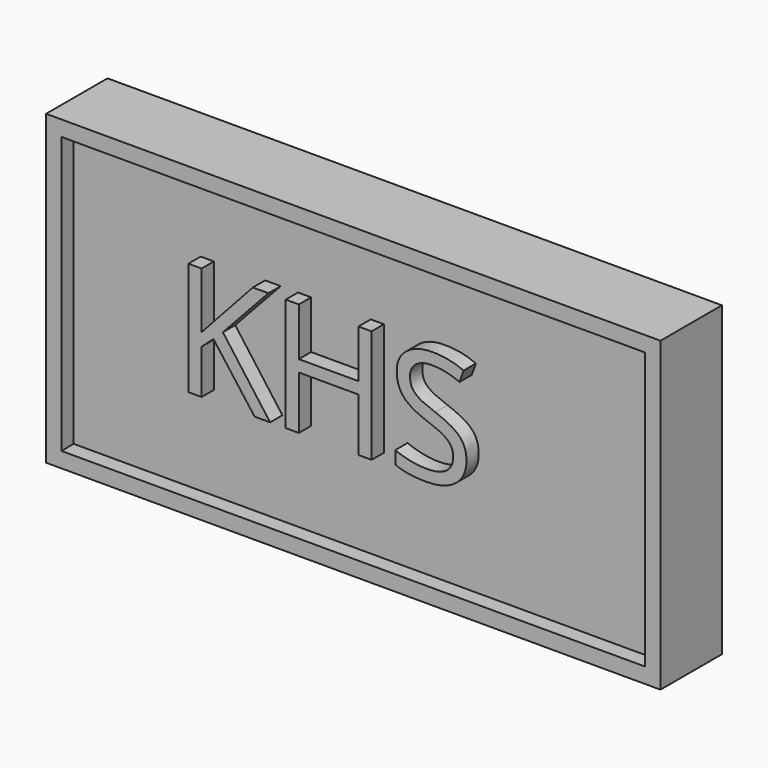
from build123d import *

# Parameters (mm, degrees)
F0_W         = 200
F0_H         = 100
F1_DEPTH     = 25
F2_W         = 190
F2_H         = 90
F3_DEPTH     = 5
F4_W         = 90
F4_H         = 50
F5_DEPTH     = 10
F6_R         = 7.5
F7_DEPTH     = 10
F8_TEXT_SIZE = 51.5888238119
F9_DEPTH     = 5


# Not quite as in the source:
# - Text() gives the source's letters only with a copy of the font that has no kerning and outlines rounded to 1/6400 em; it was checked with that copy


with BuildPart() as f1:
    # F0 (on Front) → F1 (new body)
    with BuildSketch(Plane.XZ):
        Rectangle(F0_W, F0_H)
    extrude(amount=F1_DEPTH)

    # F2 (on face) → F3 (cut)
    with BuildSketch(Plane.XZ.offset(25)):
        Rectangle(F2_W, F2_H)
    extrude(amount=-F3_DEPTH, mode=Mode.SUBTRACT)

    # F4 (on face) → F5 (join)
    with BuildSketch(Plane(origin=(0, 0, 0), x_dir=(-1, 0, 0), z_dir=(0, 1, 0))):
        Rectangle(F4_W, F4_H)
    extrude(amount=F5_DEPTH)

    # F6 (on face) → F7 (join)
    with BuildSketch(Plane(origin=(0, 10, 0), x_dir=(-1, 0, 0), z_dir=(0, 1, 0))):
        Circle(F6_R)
    extrude(amount=F7_DEPTH)

    # F8 (on face) → F9 (join)
    with BuildSketch(Plane.XZ.offset(20)):
        with Locations((-58.7308593094, -14.7128645331)):
            Text('KHS', F8_TEXT_SIZE, font='Open Sans', text_align=(TextAlign.LEFT, TextAlign.BOTTOM))
    extrude(amount=F9_DEPTH)


solid = f1.part
